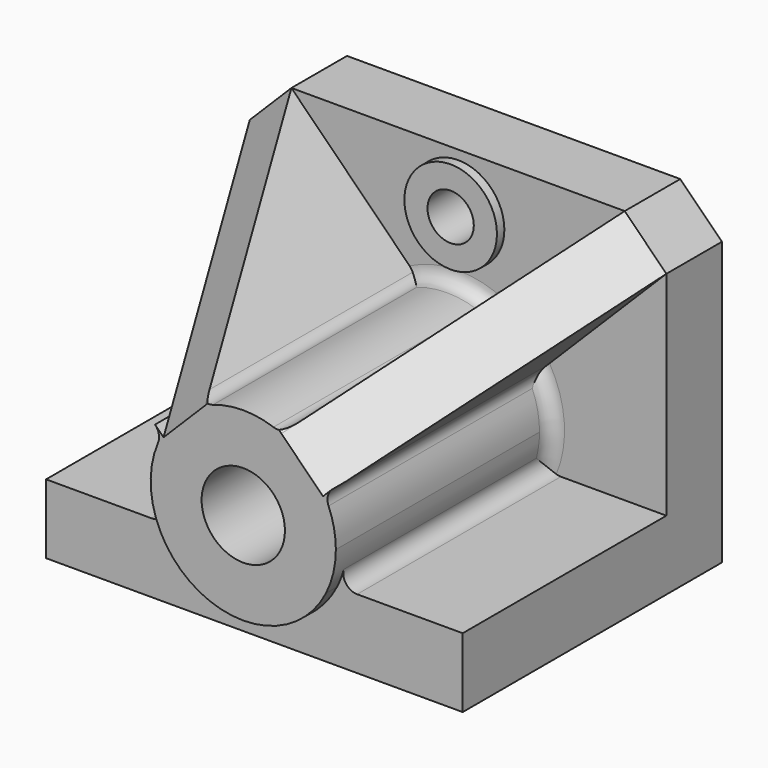
from build123d import *

# Parameters (mm, degrees)
F0_R          = 10
F1_DEPTH      = 15
F2_DEPTH      = 70
F0_R_2        = 9
F3_DEPTH      = 73
F0_R_3        = 5
F4_DEPTH      = 17
F5_SIZE2      = 9
F5_SIZE       = 9
F7_DEPTH      = 58
F9_DEPTH      = 12.7279220614
F11_DEPTH     = 12.7279220614
F12_T1_DEPTH  = 65.8575805292
F12_T6_DEPTH  = 62.9239144665
F12_T11_DEPTH = 62.9239144665
F12_T14_ANGLE = 91.5672431693
F12_T16_ANGLE = 98.292097676
F12_T18_ANGLE = 98.292097676
F12_T22_DEPTH = 67.925124519
F12_T28_DEPTH = 62.6117965858
F12_T35_DEPTH = 62.6117965858
F12_T42_DEPTH = 67.925124519
F12_T48_DEPTH = 62.6117965858
F12_T55_DEPTH = 62.6117965858


# Not quite as in the source:
# - a fillet or chamfer that OpenCascade refuses, or shapes differently, is made with other operations: its cross-section is extruded or revolved along the edge and cut away or added


with BuildPart() as f1:
    # F0 (on Front) → F1 (new body)
    with BuildSketch(Plane.XZ):
        with BuildLine():
            Line((0, 70), (0, 15))
            Line((0, 15), (27.1394289005, 15))
            ThreePointArc((27.1394289005, 15), (40.3746039083, 43.4577930659), (65, 24))
            ThreePointArc((65, 24), (64.4577930659, 19.3746039083), (62.8605710995, 15))
            Line((62.8605710995, 15), (90, 15))
            Line((90, 15), (90, 70))
            Line((90, 70), (0, 70))
        make_face()
        with Locations((45, 58)):
            Circle(F0_R, mode=Mode.SUBTRACT)
    extrude(amount=F1_DEPTH)

    # F0 (on Front) → F2 (join)
    with BuildSketch(Plane.XZ):
        with BuildLine():
            Line((0, 15), (0, 0))
            Line((0, 0), (90, 0))
            Line((90, 0), (90, 15))
            Line((90, 15), (62.8605710995, 15))
            ThreePointArc((62.8605710995, 15), (45, 4), (27.1394289005, 15))
            Line((27.1394289005, 15), (0, 15))
        make_face()
    extrude(amount=F2_DEPTH)

    # F0 (on Front) → F3 (join)
    with BuildSketch(Plane.XZ):
        with BuildLine():
            ThreePointArc((65, 24), (40.3746039083, 43.4577930659), (27.1394289005, 15))
            ThreePointArc((27.1394289005, 15), (45, 4), (62.8605710995, 15))
            ThreePointArc((62.8605710995, 15), (64.4577930659, 19.3746039083), (65, 24))
        make_face()
        with Locations((45, 24)):
            Circle(F0_R_2, mode=Mode.SUBTRACT)
    extrude(amount=F3_DEPTH)

    # F0 (on Front) → F4 (join)
    with BuildSketch(Plane.XZ):
        with Locations((45, 58)):
            Circle(F0_R)
        with Locations((45, 58)):
            Circle(F0_R_3, mode=Mode.SUBTRACT)
    extrude(amount=F4_DEPTH)

    # F5
    f5_edges = [f1.edges().sort_by_distance(p)[0] for p in [
        (90, -7.5, 70),
        (0, -7.5, 70),
    ]]
    chamfer(f5_edges, length=F5_SIZE, length2=F5_SIZE2)

    # F6 (on face) → F7 (join, through all)
    with BuildSketch(Plane.XZ.offset(15)):
        with BuildLine():
            Line((90, 61), (81, 70))
            Line((81, 70), (53.2287565553, 42.2287565553))
            ThreePointArc((53.2287565553, 42.2287565553), (58.60484202, 38.659750121), (62.5646599663, 33.5646599663))
            Line((62.5646599663, 33.5646599663), (90, 61))
        make_face()
        with BuildLine():
            Line((36.7712434447, 42.2287565553), (9, 70))
            Line((9, 70), (0, 61))
            Line((0, 61), (27.4353400337, 33.5646599663))
            ThreePointArc((27.4353400337, 33.5646599663), (31.39515798, 38.659750121), (36.7712434447, 42.2287565553))
        make_face()
    extrude(amount=F7_DEPTH)

    # F8 (on face) → F9 (cut, through all)
    with BuildSketch(Plane(origin=(5.5, 0, -5.5), x_dir=(0, -1, 0), z_dir=(-0.7071067812, 0, 0.7071067812))):
        Polygon((73, 67.4986548357), (73, 106.7731239592), (15, 106.7731239592), align=None)
    extrude(amount=-F9_DEPTH, mode=Mode.SUBTRACT)

    # F10 (on face) → F11 (cut, through all)
    with BuildSketch(Plane(origin=(39.5, 0, 39.5), x_dir=(0, 1, 0), z_dir=(0.7071067812, 0, 0.7071067812))):
        Polygon((-73, 3.859044529), (-15, 43.1335136524), (-73, 43.1335136524), align=None)
    extrude(amount=-F11_DEPTH, mode=Mode.SUBTRACT)

    # F12: fillet of radius 3 on 9 edges, made by hand

    # F12_s2 → F12_t1 (join)
    with BuildSketch(Plane.XZ.offset(4.1424194708)):
        with BuildLine():
            ThreePointArc((67.2036033112, 15), (64.821605611, 16.1762437234), (64.3074811402, 18.7826086957))
            ThreePointArc((64.3074811402, 18.7826086957), (63.6800176381, 16.8545860133), (62.8605710995, 15))
            Line((62.8605710995, 15), (67.2036033112, 15))
        make_face()
        with BuildLine():
            ThreePointArc((22.7963966888, 15), (25.178394389, 16.1762437234), (25.6925188598, 18.7826086957))
            ThreePointArc((25.6925188598, 18.7826086957), (26.3199823619, 16.8545860133), (27.1394289005, 15))
            Line((27.1394289005, 15), (22.7963966888, 15))
        make_face()
    extrude(amount=F12_T1_DEPTH)


with BuildPart() as f12_tool4:
    # F12_s5 → F12_t6 (new body)
    with BuildSketch(Plane.XZ.offset(10.0760855335)):
        with BuildLine():
            ThreePointArc((35.378550121, 43.621449879), (36.8258280598, 42.8194729683), (38.47814823, 42.9067567153))
            ThreePointArc((38.47814823, 42.9067567153), (37.6169090114, 42.5873604219), (36.7712434447, 42.2287565553))
            Line((36.7712434447, 42.2287565553), (35.378550121, 43.621449879))
        make_face()
    extrude(amount=F12_T6_DEPTH)

    split(bisect_by=Plane(origin=(-25.8358090511, -24.7411221638, 25.8358090511), x_dir=(-0.6916401802, 0.7222422455, 0), z_dir=(0.5855012217, 0.5606929988, -0.5855012217)), keep=Keep.TOP)


with BuildPart() as f1_1:
    add(f1.part)

    # F12_t3: union F12_tool4
    add(f12_tool4.part)


with BuildPart() as f12_tool9:
    # F12_s10 → F12_t11 (new body)
    with BuildSketch(Plane.XZ.offset(10.0760855335)):
        with BuildLine():
            ThreePointArc((51.52185177, 42.9067567153), (53.1741719402, 42.8194729683), (54.621449879, 43.621449879))
            Line((54.621449879, 43.621449879), (53.2287565553, 42.2287565553))
            ThreePointArc((53.2287565553, 42.2287565553), (52.3830909886, 42.5873604219), (51.52185177, 42.9067567153))
        make_face()
    extrude(amount=F12_T11_DEPTH)

    split(bisect_by=Plane(origin=(56.6888603025, -54.2869013815, 56.6888603025), x_dir=(-0.6916401802, -0.7222422455, 0), z_dir=(-0.5855012217, 0.5606929988, -0.5855012217)), keep=Keep.TOP)


with BuildPart() as f1_2:
    add(f1_1.part)

    # F12_t8: union F12_tool9
    add(f12_tool9.part)

    # F12_s13 → F12_t14 (revolve)
    with BuildSketch(Plane(origin=(33.8801327713, 0, 34.8197847954), x_dir=(0, 1, 0), z_dir=(-0.6973700085, 0, -0.7167112886))):
        with BuildLine():
            ThreePointArc((-15, -7.4848722144), (-15.8786796564, -5.3635518709), (-18, -4.4848722144))
            Line((-18, -4.4848722144), (-15, -4.4848722144))
            Line((-15, -4.4848722144), (-15, -7.4848722144))
        make_face()
    revolve(axis=Axis((45, -15, 24), (0, 1, 0)), revolution_arc=F12_T14_ANGLE)

    # F12_s15 → F12_t16 (revolve)
    with BuildSketch(Plane(origin=(14.639534214, 0, -12.2582579265), x_dir=(0, 1, 0), z_dir=(-0.7667085967, 0, 0.6419952708))):
        with BuildLine():
            ThreePointArc((-18, -67.2907935079), (-15.8786796564, -68.1694731643), (-15, -70.2907935079))
            Line((-15, -70.2907935079), (-15, -67.2907935079))
            Line((-15, -67.2907935079), (-18, -67.2907935079))
        make_face()
    revolve(axis=Axis((45, -15, 24), (0, 1, 0)), revolution_arc=F12_T16_ANGLE)

    # F12_s17 → F12_t18 (revolve)
    with BuildSketch(Plane(origin=(13.1100245291, 0, -11.708191847), x_dir=(0, 1, 0), z_dir=(0.7458581541, 0, -0.666104807))):
        with BuildLine():
            ThreePointArc((-15, 24.8753120149), (-15.8786796564, 26.9966323584), (-18, 27.8753120149))
            Line((-18, 27.8753120149), (-15, 27.8753120149))
            Line((-15, 27.8753120149), (-15, 24.8753120149))
        make_face()
    revolve(axis=Axis((45, -15, 24), (0, 1, 0)), revolution_arc=F12_T18_ANGLE)


with BuildPart() as f12_tool20:
    # F12_s21 → F12_t22 (new body)
    with BuildSketch(Plane.XZ.offset(9.6866720668)):
        with BuildLine():
            ThreePointArc((25.9325039488, 35.0674960512), (26.7555146188, 33.5214277242), (26.5749422655, 31.779283224))
            ThreePointArc((26.5749422655, 31.779283224), (26.9830125278, 32.6826356843), (27.4353400337, 33.5646599663))
            Line((27.4353400337, 33.5646599663), (25.9325039488, 35.0674960512))
        make_face()
    extrude(amount=F12_T22_DEPTH)

    split(bisect_by=Plane.XZ.offset(15), keep=Keep.BOTTOM)

    split(bisect_by=Plane(origin=(30.5, 0, 30.5), x_dir=(0, 1, 0), z_dir=(-0.7071067812, 0, -0.7071067812)), keep=Keep.TOP)


with BuildPart() as f1_3:
    add(f1_2.part)

    # F12_t19: union F12_tool20
    add(f12_tool20.part)


with BuildPart() as f12_tool26:
    # F12_s27 → F12_t28 (new body)
    with BuildSketch(Plane.XZ.offset(15)):
        with BuildLine():
            ThreePointArc((25.9325039488, 35.0674960512), (26.7555146188, 33.5214277242), (26.5749422655, 31.779283224))
            ThreePointArc((26.5749422655, 31.779283224), (26.9830125278, 32.6826356843), (27.4353400337, 33.5646599663))
            Line((27.4353400337, 33.5646599663), (25.9325039488, 35.0674960512))
        make_face()
    extrude(amount=F12_T28_DEPTH)

    split(bisect_by=Plane(origin=(-25.8358090511, -24.7411221638, 25.8358090511), x_dir=(-0.6916401802, 0.7222422455, 0), z_dir=(0.5855012217, 0.5606929988, -0.5855012217)), keep=Keep.TOP)

    split(bisect_by=Plane(origin=(30.5, 0, 30.5), x_dir=(0, 1, 0), z_dir=(-0.7071067812, 0, -0.7071067812)), keep=Keep.TOP)

    split(bisect_by=Plane.XZ.offset(73), keep=Keep.BOTTOM)


with BuildPart() as f1_4:
    add(f1_3.part)

    # F12_t25: union F12_tool26
    add(f12_tool26.part)


with BuildPart() as f12_tool33:
    # F12_s34 → F12_t35 (new body)
    with BuildSketch(Plane.XZ.offset(15)):
        with BuildLine():
            ThreePointArc((25.9325039488, 35.0674960512), (26.7555146188, 33.5214277242), (26.5749422655, 31.779283224))
            ThreePointArc((26.5749422655, 31.779283224), (26.9830125278, 32.6826356843), (27.4353400337, 33.5646599663))
            Line((27.4353400337, 33.5646599663), (25.9325039488, 35.0674960512))
        make_face()
    extrude(amount=F12_T35_DEPTH)

    split(bisect_by=Plane(origin=(-25.8358090511, -24.7411221638, 25.8358090511), x_dir=(0.6916401802, -0.7222422455, 0), z_dir=(-0.5855012217, -0.5606929988, 0.5855012217)), keep=Keep.TOP)

    split(bisect_by=Plane(origin=(30.5, 0, 30.5), x_dir=(0, 1, 0), z_dir=(-0.7071067812, 0, -0.7071067812)), keep=Keep.TOP)

    split(bisect_by=Plane.XZ.offset(73), keep=Keep.BOTTOM)


with BuildPart() as f1_5:
    add(f1_4.part)

    # F12_t32: union F12_tool33
    add(f12_tool33.part)


with BuildPart() as f12_tool40:
    # F12_s41 → F12_t42 (new body)
    with BuildSketch(Plane.XZ.offset(9.6866720668)):
        with BuildLine():
            ThreePointArc((63.4250577345, 31.779283224), (63.2444853812, 33.5214277242), (64.0674960512, 35.0674960512))
            Line((64.0674960512, 35.0674960512), (62.5646599663, 33.5646599663))
            ThreePointArc((62.5646599663, 33.5646599663), (63.0169874722, 32.6826356843), (63.4250577345, 31.779283224))
        make_face()
    extrude(amount=F12_T42_DEPTH)

    split(bisect_by=Plane(origin=(14.5, 0, -14.5), x_dir=(0, 1, 0), z_dir=(0.7071067812, 0, -0.7071067812)), keep=Keep.TOP)

    split(bisect_by=Plane.XZ.offset(15), keep=Keep.BOTTOM)


with BuildPart() as f1_6:
    add(f1_5.part)

    # F12_t39: union F12_tool40
    add(f12_tool40.part)


with BuildPart() as f12_tool46:
    # F12_s47 → F12_t48 (new body)
    with BuildSketch(Plane.XZ.offset(15)):
        with BuildLine():
            ThreePointArc((63.4250577345, 31.779283224), (63.2444853812, 33.5214277242), (64.0674960512, 35.0674960512))
            Line((64.0674960512, 35.0674960512), (62.5646599663, 33.5646599663))
            ThreePointArc((62.5646599663, 33.5646599663), (63.0169874722, 32.6826356843), (63.4250577345, 31.779283224))
        make_face()
    extrude(amount=F12_T48_DEPTH)

    split(bisect_by=Plane.XZ.offset(73), keep=Keep.BOTTOM)

    split(bisect_by=Plane(origin=(14.5, 0, -14.5), x_dir=(0, 1, 0), z_dir=(0.7071067812, 0, -0.7071067812)), keep=Keep.TOP)

    split(bisect_by=Plane(origin=(56.6888603025, -54.2869013815, 56.6888603025), x_dir=(-0.6916401802, -0.7222422455, 0), z_dir=(-0.5855012217, 0.5606929988, -0.5855012217)), keep=Keep.TOP)


with BuildPart() as f1_7:
    add(f1_6.part)

    # F12_t45: union F12_tool46
    add(f12_tool46.part)


with BuildPart() as f12_tool53:
    # F12_s54 → F12_t55 (new body)
    with BuildSketch(Plane.XZ.offset(15)):
        with BuildLine():
            ThreePointArc((63.4250577345, 31.779283224), (63.2444853812, 33.5214277242), (64.0674960512, 35.0674960512))
            Line((64.0674960512, 35.0674960512), (62.5646599663, 33.5646599663))
            ThreePointArc((62.5646599663, 33.5646599663), (63.0169874722, 32.6826356843), (63.4250577345, 31.779283224))
        make_face()
    extrude(amount=F12_T55_DEPTH)

    split(bisect_by=Plane.XZ.offset(73), keep=Keep.BOTTOM)

    split(bisect_by=Plane(origin=(14.5, 0, -14.5), x_dir=(0, 1, 0), z_dir=(0.7071067812, 0, -0.7071067812)), keep=Keep.TOP)

    split(bisect_by=Plane(origin=(56.6888603025, -54.2869013815, 56.6888603025), x_dir=(0.6916401802, 0.7222422455, 0), z_dir=(0.5855012217, -0.5606929988, 0.5855012217)), keep=Keep.TOP)


with BuildPart() as f1_8:
    add(f1_7.part)

    # F12_t52: union F12_tool53
    add(f12_tool53.part)


solid = f1_8.part
